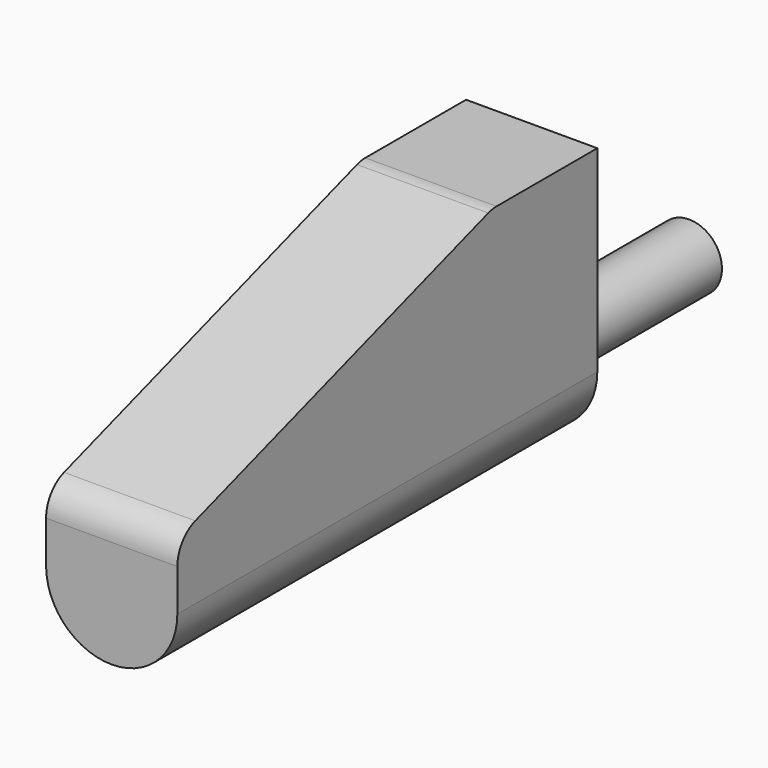
from build123d import *

# Parameters (mm, degrees)
F1_DEPTH = 20
F2_R     = 9.99999
F3_R     = 5
F4_DEPTH = 30


# Not quite as in the source:
# - a fillet or chamfer is up to 0.001 mm smaller than in the source, because OpenCascade refuses the exact size


with BuildPart() as f1:
    # F0 (on Right) → F1 (new body)
    with BuildSketch(Plane.YZ):
        with BuildLine():
            Line((-80, 0), (0, 0))
            Line((0, 0), (0, 40))
            Line((0, 40), (-19.1886116992, 40))
            ThreePointArc((-19.1886116992, 40), (-19.9895229142, 39.9354372882), (-20.7697505292, 39.7434164903))
            Line((-20.7697505292, 39.7434164903), (-76.5811388301, 21.13962039))
            ThreePointArc((-76.5811388301, 21.13962039), (-79.0562109259, 19.319755323), (-80, 16.3962038997))
            Line((-80, 16.3962038997), (-80, 0))
        make_face()
    extrude(amount=F1_DEPTH)

    # F2 (radius 10 in the source; OpenCascade refuses exactly that, so slightly less here)
    f2_edges = [f1.edges().sort_by_distance(p)[0] for p in [
        (20, -40, 0),
        (0, -40, 0),
    ]]
    fillet(f2_edges, radius=F2_R)

    # F3 (on face) → F4 (join)
    with BuildSketch(Plane(origin=(0, 0, 0), x_dir=(-1, 0, 0), z_dir=(0, 1, 0))):
        with Locations((-10, 10)):
            Circle(F3_R)
    extrude(amount=F4_DEPTH)


solid = f1.part
